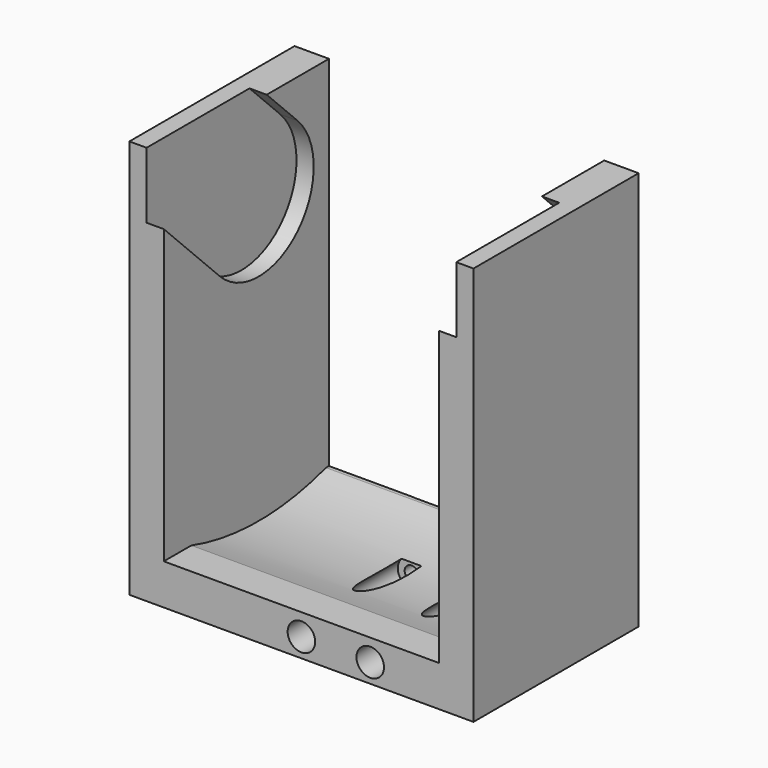
from build123d import *

# Parameters (mm, degrees)
F1_DEPTH       = 15.0114
F2_W           = 12.7
F2_H           = 76.2
F3_DEPTH       = 147.32
F4_R           = 2.54
F5_DEPTH       = 76.201
F7_DEPTH       = 6.35
F8_R           = 5.08
F9_DEPTH       = 50.8
F11_DEPTH      = 6.35
F11_DEPTH_BACK = 82.55
F15_DEPTH      = 50.8
F16_W          = 63.9064
F16_H          = 15.0114
F17_DEPTH      = 0.1016


# Not quite as in the source:
# - a pattern or mirror of a feature is missing from the dataset's text; its kind, count and spacing are read off the source's solid


with BuildPart() as f1:
    # F0 (on Top) → F1 (new body)
    with BuildSketch(Plane.XY):
        Polygon((-38.1, -38.1), (38.1, -38.1), (38.1, 38.1), (-38.1, 38.1), (-63.5, 38.1), (-63.5, -38.1), align=None)
    extrude(amount=F1_DEPTH)

    # F2 (on Top) → F3 (join)
    with BuildSketch(Plane.XY):
        with Locations((-69.85, 0)):
            Rectangle(F2_W, F2_H)
        with Locations((44.45, 0)):
            Rectangle(F2_W, F2_H)
    extrude(amount=F3_DEPTH)

    # F4 (on face) → F5 (cut, through all)
    with BuildSketch(Plane.XZ.offset(38.1)):
        with Locations((-12.7, 7.0104)):
            Circle(F4_R)
        with Locations((12.7, 7.0104)):
            Circle(F4_R)
    extrude(amount=-F5_DEPTH, mode=Mode.SUBTRACT)

    # F6 (on face) → F7 (cut)
    with BuildSketch(Plane(origin=(0, 38.1, 0), x_dir=(-1, 0, 0), z_dir=(0, 1, 0))):
        Polygon((-7.9502, 7.0104), (-10.3251, 11.1238474629), (-15.0749, 11.1238474629), (-17.4498, 7.0104), (-15.0749, 2.8969525371), (-10.3251, 2.8969525371), align=None)
        Polygon((17.4498, 7.0104), (15.0749, 11.1238474629), (10.3251, 11.1238474629), (7.9502, 7.0104), (10.3251, 2.8969525371), (15.0749, 2.8969525371), align=None)
    extrude(amount=-F7_DEPTH, mode=Mode.SUBTRACT)

    # F8 (on face) → F9 (cut)
    with BuildSketch(Plane.XZ.offset(38.1)):
        with Locations((-12.7, 7.0104)):
            Circle(F8_R)
        with Locations((12.7, 7.0104)):
            Circle(F8_R)
    extrude(amount=-F9_DEPTH, mode=Mode.SUBTRACT)

    # F10 (on face) → F11 (cut, two sides)
    with BuildSketch(Plane.YZ.offset(-63.5)) as f11_sk:
        with BuildLine():
            Line((-38.1, 122.9614), (-12.2968071525, 97.1582071525))
            ThreePointArc((-12.2968071525, 97.1582071525), (23.6242173318, 97.1582071525), (23.6242173318, 133.0792316368))
            Line((23.6242173318, 133.0792316368), (9.3834489686, 147.32))
            Line((9.3834489686, 147.32), (-38.1, 147.32))
            Line((-38.1, 147.32), (-38.1, 122.9614))
        make_face()
    f11 = extrude(amount=-F11_DEPTH, mode=Mode.SUBTRACT) + extrude(f11_sk.sketch, amount=F11_DEPTH_BACK, mode=Mode.SUBTRACT)

    # F11_copies: F11 across plane
    add(f11.mirror(Plane(origin=(-12.7, 0, 0), x_dir=(0, 0, 1), z_dir=(1, 0, 0))), mode=Mode.SUBTRACT)

    # F14 (on line) → F15 (cut, symmetric)
    with BuildSketch(Plane(origin=(-12.7, 0, 0), x_dir=(0, -1, 0), z_dir=(-1, 0, 0))):
        with BuildLine():
            Line((25.4, 15.0114), (-36.7274101792, 15.0114))
            ThreePointArc((-36.7274101792, 15.0114), (-5.6637050896, 10.3025509364), (25.4, 15.0114))
        make_face()
    extrude(amount=F15_DEPTH, both=True, mode=Mode.SUBTRACT)

    # F16 (on face) → F17 (cut)
    with BuildSketch(Plane(origin=(0, 38.1, 0), x_dir=(-1, 0, 0), z_dir=(0, 1, 0))):
        with Locations((0, 7.5057)):
            Rectangle(F16_W, F16_H)
    extrude(amount=-F17_DEPTH, mode=Mode.SUBTRACT)


solid = f1.part
